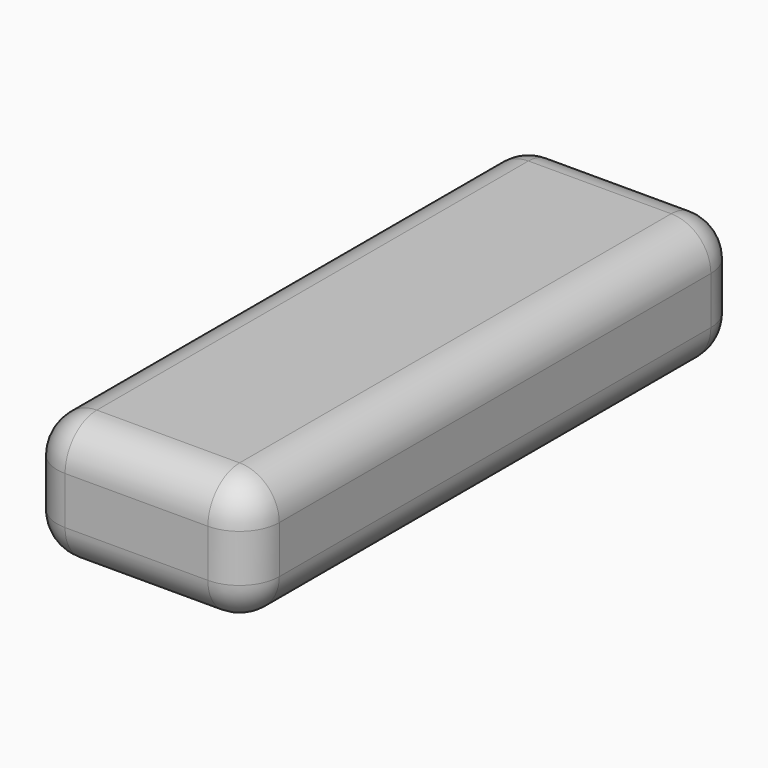
from build123d import *

# Parameters (mm, degrees)
F0_W         = 28
F0_H         = 16
F1_DEPTH     = 78
F2_R         = 2.2016502053
F4_DEPTH     = 67.8
F5_R         = 1.5264270503
F6_DEPTH     = 10.6
F3_R         = 8.2210139084
F7_DEPTH     = 5.5
F8_T1_DEPTH  = 68
F8_T3_DEPTH  = 18
F8_T5_DEPTH  = 6
F8_S9_W      = 5
F8_S9_H      = 5
F8_T10_DEPTH = 5
F8_S15_W     = 5
F8_S15_H     = 5
F8_T16_DEPTH = 5
F8_S21_W     = 5
F8_S21_H     = 5
F8_T22_DEPTH = 5
F8_S27_W     = 5
F8_S27_H     = 5
F8_T28_DEPTH = 5
F8_S33_W     = 5
F8_S33_H     = 5
F8_T34_DEPTH = 5
F8_S39_W     = 5
F8_S39_H     = 5
F8_T40_DEPTH = 5
F8_S45_W     = 5
F8_S45_H     = 5
F8_T46_DEPTH = 5
F8_S51_W     = 5
F8_S51_H     = 5
F8_T52_DEPTH = 5


# Not quite as in the source:
# - a fillet or chamfer that OpenCascade refuses, or shapes differently, is made with other operations: its cross-section is extruded or revolved along the edge and cut away or added


with BuildPart() as f1:
    # F0 (on Front) → F1 (new body)
    with BuildSketch(Plane.XZ):
        Rectangle(F0_W, F0_H)
    extrude(amount=F1_DEPTH)

    # F2 (on face) → F4 (cut)
    with BuildSketch(Plane(origin=(0, 0, 0), x_dir=(-1, 0, 0), z_dir=(0, 1, 0))):
        Circle(F2_R)
    extrude(amount=-F4_DEPTH, mode=Mode.SUBTRACT)

    # F5 (on face) → F6 (cut)
    with BuildSketch(Plane(origin=(0, 0, -8), x_dir=(1, 0, 0), z_dir=(0, 0, -1))):
        with Locations((0, 66.9171065092)):
            Circle(F5_R)
    extrude(amount=-F6_DEPTH, mode=Mode.SUBTRACT)

    # F3 (on face) → F7 (cut)
    with BuildSketch(Plane(origin=(0, 0, -8), x_dir=(1, 0, 0), z_dir=(0, 0, -1))):
        with Locations((0, 66.784389317)):
            Circle(F3_R)
    extrude(amount=-F7_DEPTH, mode=Mode.SUBTRACT)

    # F8: fillet of radius 5 on 12 edges, made by hand

    # F8_s2 → F8_t1 (cut)
    with BuildSketch(Plane.XZ.offset(5)):
        with BuildLine():
            ThreePointArc((-14, -3), (-12.5355339059, -6.5355339059), (-9, -8))
            Line((-9, -8), (-14, -8))
            Line((-14, -8), (-14, -3))
        make_face()
        with BuildLine():
            ThreePointArc((14, -3), (12.5355339059, -6.5355339059), (9, -8))
            Line((9, -8), (14, -8))
            Line((14, -8), (14, -3))
        make_face()
        with BuildLine():
            ThreePointArc((9, 8), (12.5355339059, 6.5355339059), (14, 3))
            Line((14, 3), (14, 8))
            Line((14, 8), (9, 8))
        make_face()
        with BuildLine():
            ThreePointArc((-9, 8), (-12.5355339059, 6.5355339059), (-14, 3))
            Line((-14, 3), (-14, 8))
            Line((-14, 8), (-9, 8))
        make_face()
    extrude(amount=F8_T1_DEPTH, mode=Mode.SUBTRACT)

    # F8_s4 → F8_t3 (cut)
    with BuildSketch(Plane.YZ.offset(-9)):
        with BuildLine():
            ThreePointArc((-78, -3), (-76.5355339059, -6.5355339059), (-73, -8))
            Line((-73, -8), (-78, -8))
            Line((-78, -8), (-78, -3))
        make_face()
        with BuildLine():
            ThreePointArc((0, -3), (-1.4644660941, -6.5355339059), (-5, -8))
            Line((-5, -8), (0, -8))
            Line((0, -8), (0, -3))
        make_face()
        with BuildLine():
            ThreePointArc((-5, 8), (-1.4644660941, 6.5355339059), (0, 3))
            Line((0, 3), (0, 8))
            Line((0, 8), (-5, 8))
        make_face()
        with BuildLine():
            ThreePointArc((-73, 8), (-76.5355339059, 6.5355339059), (-78, 3))
            Line((-78, 3), (-78, 8))
            Line((-78, 8), (-73, 8))
        make_face()
    extrude(amount=F8_T3_DEPTH, mode=Mode.SUBTRACT)

    # F8_s6 → F8_t5 (cut)
    with BuildSketch(Plane.XY.offset(-3)):
        with BuildLine():
            ThreePointArc((14, -73), (12.5355339059, -76.5355339059), (9, -78))
            Line((9, -78), (14, -78))
            Line((14, -78), (14, -73))
        make_face()
        with BuildLine():
            ThreePointArc((-14, -73), (-12.5355339059, -76.5355339059), (-9, -78))
            Line((-9, -78), (-14, -78))
            Line((-14, -78), (-14, -73))
        make_face()
        with BuildLine():
            ThreePointArc((-14, -5), (-12.5355339059, -1.4644660941), (-9, 0))
            Line((-9, 0), (-14, 0))
            Line((-14, 0), (-14, -5))
        make_face()
        with BuildLine():
            ThreePointArc((14, -5), (12.5355339059, -1.4644660941), (9, 0))
            Line((9, 0), (14, 0))
            Line((14, 0), (14, -5))
        make_face()
    extrude(amount=F8_T5_DEPTH, mode=Mode.SUBTRACT)


with BuildPart() as f8_tool8:
    # F8_s9 → F8_t10 (new body)
    with BuildSketch(Plane.YZ.offset(-9)):
        with Locations((-2.5, -5.5)):
            Rectangle(F8_S9_W, F8_S9_H)
    extrude(amount=-F8_T10_DEPTH)

    # F8_s11 → F8_t12 (revolve, cut)
    with BuildSketch(Plane(origin=(-9, -5, -3), x_dir=(0, -0.7071067812, 0.7071067812), z_dir=(0, -0.7071067812, -0.7071067812))):
        with BuildLine():
            ThreePointArc((0, -5), (5, 0), (0, 5))
            Line((0, 5), (0, -5))
        make_face()
    revolve(axis=Axis((-9, -5, -3), (-1, 0, 0)), mode=Mode.SUBTRACT)


with BuildPart() as f1_1:
    add(f1.part)

    # F8_t7: cut F8_tool8
    add(f8_tool8.part, mode=Mode.SUBTRACT)


with BuildPart() as f8_tool14:
    # F8_s15 → F8_t16 (new body)
    with BuildSketch(Plane.YZ.offset(-9)):
        with Locations((-75.5, -5.5)):
            Rectangle(F8_S15_W, F8_S15_H)
    extrude(amount=-F8_T16_DEPTH)

    # F8_s17 → F8_t18 (revolve, cut)
    with BuildSketch(Plane(origin=(-9, -73, -3), x_dir=(0, 0.7071067812, 0.7071067812), z_dir=(0, -0.7071067812, 0.7071067812))):
        with BuildLine():
            ThreePointArc((0, -5), (5, 0), (0, 5))
            Line((0, 5), (0, -5))
        make_face()
    revolve(axis=Axis((-9, -73, -3), (-1, 0, 0)), mode=Mode.SUBTRACT)


with BuildPart() as f1_2:
    add(f1_1.part)

    # F8_t13: cut F8_tool14
    add(f8_tool14.part, mode=Mode.SUBTRACT)


with BuildPart() as f8_tool20:
    # F8_s21 → F8_t22 (new body)
    with BuildSketch(Plane.YZ.offset(9)):
        with Locations((-75.5, -5.5)):
            Rectangle(F8_S21_W, F8_S21_H)
    extrude(amount=F8_T22_DEPTH)

    # F8_s23 → F8_t24 (revolve, cut)
    with BuildSketch(Plane(origin=(9, -73, -3), x_dir=(0, 0.7071067812, 0.7071067812), z_dir=(0, 0.7071067812, -0.7071067812))):
        with BuildLine():
            ThreePointArc((0, -5), (5, 0), (0, 5))
            Line((0, 5), (0, -5))
        make_face()
    revolve(axis=Axis((9, -73, -3), (1, 0, 0)), mode=Mode.SUBTRACT)


with BuildPart() as f1_3:
    add(f1_2.part)

    # F8_t19: cut F8_tool20
    add(f8_tool20.part, mode=Mode.SUBTRACT)


with BuildPart() as f8_tool26:
    # F8_s27 → F8_t28 (new body)
    with BuildSketch(Plane.YZ.offset(9)):
        with Locations((-2.5, -5.5)):
            Rectangle(F8_S27_W, F8_S27_H)
    extrude(amount=F8_T28_DEPTH)

    # F8_s29 → F8_t30 (revolve, cut)
    with BuildSketch(Plane(origin=(9, -5, -3), x_dir=(0, -0.7071067812, 0.7071067812), z_dir=(0, 0.7071067812, 0.7071067812))):
        with BuildLine():
            ThreePointArc((0, -5), (5, 0), (0, 5))
            Line((0, 5), (0, -5))
        make_face()
    revolve(axis=Axis((9, -5, -3), (1, 0, 0)), mode=Mode.SUBTRACT)


with BuildPart() as f1_4:
    add(f1_3.part)

    # F8_t25: cut F8_tool26
    add(f8_tool26.part, mode=Mode.SUBTRACT)


with BuildPart() as f8_tool32:
    # F8_s33 → F8_t34 (new body)
    with BuildSketch(Plane.XY.offset(3)):
        with Locations((11.5, -2.5)):
            Rectangle(F8_S33_W, F8_S33_H)
    extrude(amount=F8_T34_DEPTH)

    # F8_s35 → F8_t36 (revolve, cut)
    with BuildSketch(Plane(origin=(9, -5, 3), x_dir=(-0.7071067812, -0.7071067812, 0), z_dir=(-0.7071067812, 0.7071067812, 0))):
        with BuildLine():
            ThreePointArc((0, -5), (5, 0), (0, 5))
            Line((0, 5), (0, -5))
        make_face()
    revolve(axis=Axis((9, -5, 3), (0, 0, 1)), mode=Mode.SUBTRACT)


with BuildPart() as f1_5:
    add(f1_4.part)

    # F8_t31: cut F8_tool32
    add(f8_tool32.part, mode=Mode.SUBTRACT)


with BuildPart() as f8_tool38:
    # F8_s39 → F8_t40 (new body)
    with BuildSketch(Plane.XY.offset(3)):
        with Locations((-11.5, -2.5)):
            Rectangle(F8_S39_W, F8_S39_H)
    extrude(amount=F8_T40_DEPTH)

    # F8_s41 → F8_t42 (revolve, cut)
    with BuildSketch(Plane(origin=(-9, -5, 3), x_dir=(0.7071067812, -0.7071067812, 0), z_dir=(-0.7071067812, -0.7071067812, 0))):
        with BuildLine():
            ThreePointArc((0, -5), (5, 0), (0, 5))
            Line((0, 5), (0, -5))
        make_face()
    revolve(axis=Axis((-9, -5, 3), (0, 0, 1)), mode=Mode.SUBTRACT)


with BuildPart() as f1_6:
    add(f1_5.part)

    # F8_t37: cut F8_tool38
    add(f8_tool38.part, mode=Mode.SUBTRACT)


with BuildPart() as f8_tool44:
    # F8_s45 → F8_t46 (new body)
    with BuildSketch(Plane.XY.offset(3)):
        with Locations((11.5, -75.5)):
            Rectangle(F8_S45_W, F8_S45_H)
    extrude(amount=F8_T46_DEPTH)

    # F8_s47 → F8_t48 (revolve, cut)
    with BuildSketch(Plane(origin=(9, -73, 3), x_dir=(-0.7071067812, 0.7071067812, 0), z_dir=(0.7071067812, 0.7071067812, 0))):
        with BuildLine():
            ThreePointArc((0, -5), (5, 0), (0, 5))
            Line((0, 5), (0, -5))
        make_face()
    revolve(axis=Axis((9, -73, 3), (0, 0, 1)), mode=Mode.SUBTRACT)


with BuildPart() as f1_7:
    add(f1_6.part)

    # F8_t43: cut F8_tool44
    add(f8_tool44.part, mode=Mode.SUBTRACT)


with BuildPart() as f8_tool50:
    # F8_s51 → F8_t52 (new body)
    with BuildSketch(Plane.XY.offset(3)):
        with Locations((-11.5, -75.5)):
            Rectangle(F8_S51_W, F8_S51_H)
    extrude(amount=F8_T52_DEPTH)

    # F8_s53 → F8_t54 (revolve, cut)
    with BuildSketch(Plane(origin=(-9, -73, 3), x_dir=(0.7071067812, 0.7071067812, 0), z_dir=(0.7071067812, -0.7071067812, 0))):
        with BuildLine():
            ThreePointArc((0, -5), (5, 0), (0, 5))
            Line((0, 5), (0, -5))
        make_face()
    revolve(axis=Axis((-9, -73, 3), (0, 0, 1)), mode=Mode.SUBTRACT)


with BuildPart() as f1_8:
    add(f1_7.part)

    # F8_t49: cut F8_tool50
    add(f8_tool50.part, mode=Mode.SUBTRACT)


solid = f1_8.part
